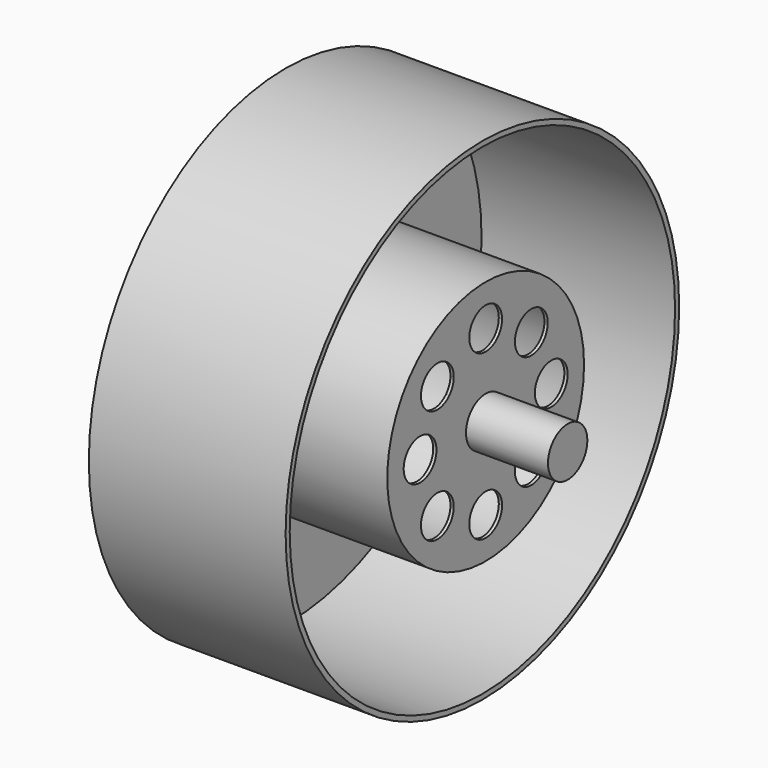
from build123d import *

# Parameters (mm, degrees)
F0_R      = 19.05
F1_DEPTH  = 15.24
F2_R      = 18.653125
F3_DEPTH  = 14.986
F4_R      = 9.525
F5_DEPTH  = 15.24
F7_R      = 1.5875
F8_DEPTH  = 2.54
F9_R      = 8.89
F10_DEPTH = 15.24
F11_R     = 1.905
F12_DEPTH = 6.35


# Not quite as in the source:
# - a feature names something its author has since deleted; it is built from what else it names


with BuildPart() as f1:
    # F0 (on Right) → F1 (new body)
    with BuildSketch(Plane.YZ):
        Circle(F0_R)
    extrude(amount=F1_DEPTH)

    # F2 (on face) → F3 (cut)
    with BuildSketch(Plane.YZ.offset(15.24)):
        Circle(F2_R)
    extrude(amount=-F3_DEPTH, mode=Mode.SUBTRACT)

    # F4 (on face) → F5 (join)
    with BuildSketch(Plane.YZ.offset(0.254)):
        Circle(F4_R)
    extrude(amount=F5_DEPTH)

    # F7 (on face) → F8 (cut)
    with BuildSketch(Plane.YZ.offset(15.494)):
        with BuildLine():
            ThreePointArc((1.5875, 6.35), (-1.1225320151, 7.4725320151), (0, 4.7625))
            ThreePointArc((0, 4.7625), (1.1225320151, 5.2274679849), (1.5875, 6.35))
        make_face()
        with BuildLine():
            ThreePointArc((7.9375, 0), (6.35, 1.5875), (4.7625, 0))
            ThreePointArc((4.7625, 0), (6.35, -1.5875), (7.9375, 0))
        make_face()
        with BuildLine():
            ThreePointArc((1.5875, -6.35), (1.1225320151, -5.2274679849), (0, -4.7625))
            ThreePointArc((0, -4.7625), (-1.1225320151, -7.4725320151), (1.5875, -6.35))
        make_face()
        with Locations((-6.35, 0)):
            Circle(F7_R)
        with BuildLine():
            ThreePointArc((6.0059587639, 4.2942080269), (3.8214214188, 5.7651610032), (3.2800341547, 3.187796865))
            ThreePointArc((3.2800341547, 3.187796865), (5.015496109, 2.8232550506), (6.0059587639, 4.2942080269))
        make_face()
        with BuildLine():
            ThreePointArc((6.0059587639, -4.5463046331), (5.0364104329, -3.0840146534), (3.312047602, -3.4078800239))
            ThreePointArc((3.312047602, -3.4078800239), (3.8005070949, -6.0085946128), (6.0059587639, -4.5463046331))
        make_face()
        with BuildLine():
            ThreePointArc((-3.0903496579, -4.5463046331), (-3.2068966816, -3.949267288), (-3.5394250487, -3.4398934712))
            ThreePointArc((-3.5394250487, -3.4398934712), (-6.1488026342, -5.1433419782), (-3.0903496579, -4.5463046331))
        make_face()
        with BuildLine():
            ThreePointArc((-3.0903496579, 4.2942080269), (-6.157153182, 4.8702439055), (-3.5083872434, 3.2206560202))
            ThreePointArc((-3.5083872434, 3.2206560202), (-3.1985461338, 3.7181721482), (-3.0903496579, 4.2942080269))
        make_face()
    extrude(amount=-F8_DEPTH, mode=Mode.SUBTRACT)

    # F9 (on face) → F10 (cut)
    with BuildSketch(Plane(origin=(0, 0, 0), x_dir=(0, -1, 0), z_dir=(-1, 0, 0))):
        Circle(F9_R)
    extrude(amount=-F10_DEPTH, mode=Mode.SUBTRACT)

    # F11 (on face) → F12 (join)
    with BuildSketch(Plane.YZ.offset(15.494)):
        Circle(F11_R)
    extrude(amount=F12_DEPTH)


solid = f1.part
